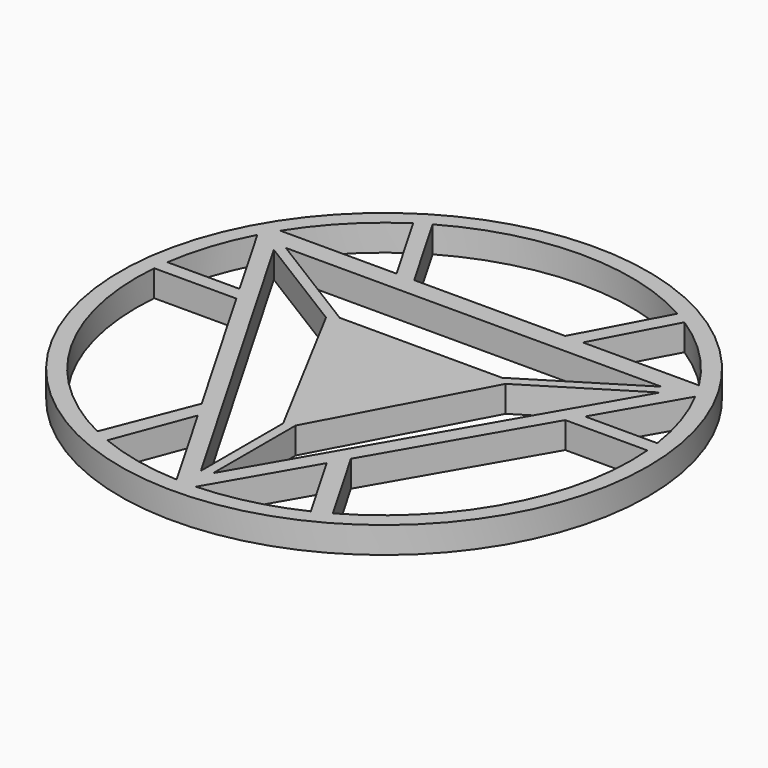
from build123d import *

# Parameters (mm, degrees)
F0_R     = 50.8
F1_DEPTH = 5.08


# Not quite as in the source:
# - a feature names something its author has since deleted; it is built from what else it names


with BuildPart() as f1:
    # F0 (on Top) → F1 (new body)
    with BuildSketch(Plane.XY):
        Circle(F0_R)
        with BuildLine():
            Line((-17.9742814731, -44.1029004775), (-12.4049825801, -29.3139399042))
            Line((-12.4049825801, -29.3139399042), (-1.8539284107, -47.5889017991))
            ThreePointArc((-1.8539284107, -47.5889017991), (-10.066157564, -46.549039699), (-17.9742814731, -44.1029004775))
        make_face(mode=Mode.SUBTRACT)
        with BuildLine():
            ThreePointArc((-20.9620816677, -42.7636733356), (-41.4419156704, -23.4671738939), (-47.4549141022, 4.0214117617))
            Line((-47.4549141022, 4.0214117617), (-31.651156838, 4.0214117617))
            Line((-31.651156838, 4.0214117617), (-14.3567544825, -25.9333718046))
            Line((-14.3567544825, -25.9333718046), (-20.9620816677, -42.7636733356))
        make_face(mode=Mode.SUBTRACT)
        Polygon((-0.7916404097, -43.0788385891), (-37.1806461747, 19.9487682329), (-17.281252241, 7.6313526128), (-0.7916404097, -23.293502324), align=None, mode=Mode.SUBTRACT)
        with BuildLine():
            ThreePointArc((20.3423780674, -43.061912168), (11.3266241262, -46.2584933921), (1.8539284107, -47.5889017991))
            Line((1.8539284107, -47.5889017991), (12.4049825801, -29.3139399042))
            Line((12.4049825801, -29.3139399042), (20.3423780674, -43.061912168))
        make_face(mode=Mode.SUBTRACT)
        Polygon((17.2735304892, 7.6168711285), (37.1719298571, 19.9336711278), (1.1133595903, -42.5216046224), (1.1133595903, -22.6901455503), align=None, mode=Mode.SUBTRACT)
        with BuildLine():
            Line((14.3567544825, -25.9333718046), (31.651156838, 4.0214117617))
            Line((31.651156838, 4.0214117617), (47.4549141022, 4.0214117617))
            ThreePointArc((47.4549141022, 4.0214117617), (42.0897424453, -22.2843937743), (23.3490930586, -41.5085590974))
            Line((23.3490930586, -41.5085590974), (14.3567544825, -25.9333718046))
        make_face(mode=Mode.SUBTRACT)
        with BuildLine():
            ThreePointArc((-47.1383927866, 6.7906222465), (-45.2983646948, 14.7036995676), (-42.1401621016, 22.1889017991))
            Line((-42.1401621016, 22.1889017991), (-33.2499612568, 6.7906222465))
            Line((-33.2499612568, 6.7906222465), (-47.1383927866, 6.7906222465))
        make_face(mode=Mode.SUBTRACT)
        with BuildLine():
            Line((-17.9263273651, 25.4), (-40.2862336909, 25.4))
            ThreePointArc((-40.2862336909, 25.4), (-34.0178257765, 33.3305888703), (-26.2168031881, 39.7595253442))
            Line((-26.2168031881, 39.7595253442), (-17.9263273651, 25.4))
        make_face(mode=Mode.SUBTRACT)
        with BuildLine():
            ThreePointArc((-23.7093258464, 41.3038556664), (-0.3049103548, 47.6240239236), (23.1785122433, 41.6040526293))
            Line((23.1785122433, 41.6040526293), (14.5382603004, 25.4))
            Line((14.5382603004, 25.4), (-14.5272304963, 25.4))
            Line((-14.5272304963, 25.4), (-23.7093258464, 41.3038556664))
        make_face(mode=Mode.SUBTRACT)
        Polygon((-15.6162167432, 8.8411357684), (-36.1336946584, 21.5411357684), (36.1493684604, 21.5411357684), (15.6318905452, 8.8411357684), align=None, mode=Mode.SUBTRACT)
        with BuildLine():
            Line((47.1383927866, 6.7906222465), (33.2499612568, 6.7906222465))
            Line((33.2499612568, 6.7906222465), (42.1401621016, 22.1889017991))
            ThreePointArc((42.1401621016, 22.1889017991), (45.2983646948, 14.7036995676), (47.1383927866, 6.7906222465))
        make_face(mode=Mode.SUBTRACT)
        with BuildLine():
            Line((40.2862336909, 25.4), (17.9263273651, 25.4))
            Line((17.9263273651, 25.4), (25.7463457142, 40.065774763))
            ThreePointArc((25.7463457142, 40.065774763), (33.8208016326, 33.5304936129), (40.2862336909, 25.4))
        make_face(mode=Mode.SUBTRACT)
    extrude(amount=F1_DEPTH)


solid = f1.part
